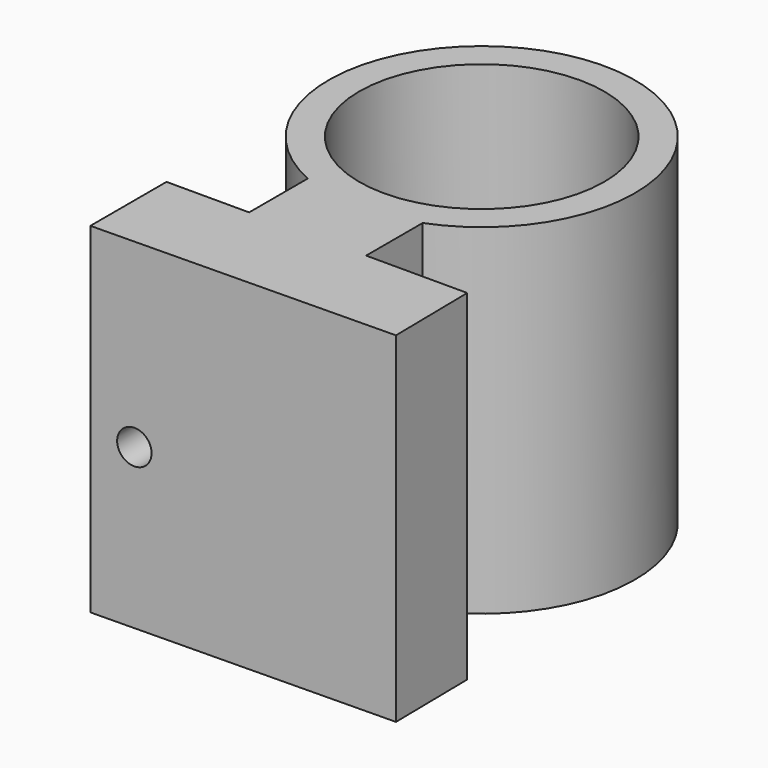
from build123d import *

# Parameters (mm, degrees)
F1_DEPTH = 38.1
F2_R     = 13.716
F3_DEPTH = 50.292
F4_R     = 1.905
F5_DEPTH = 25.4


# Not quite as in the source:
# - a feature names something its author has since deleted; it is built from what else it names


with BuildPart() as f1:
    # F0 (on Top) → F1 (new body)
    with BuildSketch(Plane.XY):
        with BuildLine():
            ThreePointArc((6.1794301228, -15.9926754597), (14.1403209733, -9.6954807912), (17.145, 0))
            ThreePointArc((17.145, 0), (-9.3627294025, 14.3628104191), (-6.9191963412, -15.6868016814))
            ThreePointArc((-6.9191963412, -15.6868016814), (-0.4002539276, -17.1403273537), (6.1794301228, -15.9926754597))
        make_face()
        with BuildLine():
            ThreePointArc((6.1794301228, -15.9926754597), (-0.4002539276, -17.1403273537), (-6.9191963412, -15.6868016814))
            Line((-6.9191963412, -15.6868016814), (-6.9191963412, -23.9002238959))
            Line((-6.9191963412, -23.9002238959), (-16.1695149392, -23.9002238959))
            Line((-16.1695149392, -23.9002238959), (-16.1695149392, -34.5569381251))
            Line((-16.1695149392, -34.5569381251), (17.6482256417, -34.0591232702))
            Line((17.6482256417, -34.0591232702), (17.4986813217, -23.9002238959))
            Line((17.4986813217, -23.9002238959), (6.1794301228, -23.9002238959))
            Line((6.1794301228, -23.9002238959), (6.1794301228, -21.5747152004))
            Line((6.1794301228, -21.5747152004), (6.1794301228, -15.9926754597))
        make_face()
    extrude(amount=F1_DEPTH)

    # F2 (on face) → F3 (cut)
    with BuildSketch(Plane.XY.offset(38.1)):
        Circle(F2_R)
    extrude(amount=-F3_DEPTH, mode=Mode.SUBTRACT)

    # F4 (on face) → F5 (cut)
    with BuildSketch(Plane(origin=(0, -23.9002238959, 0), x_dir=(-1, 0, 0), z_dir=(0, 1, 0))):
        with Locations((11.3007957116, 17.8492013365)):
            Circle(F4_R)
    extrude(amount=-F5_DEPTH, mode=Mode.SUBTRACT)


solid = f1.part
